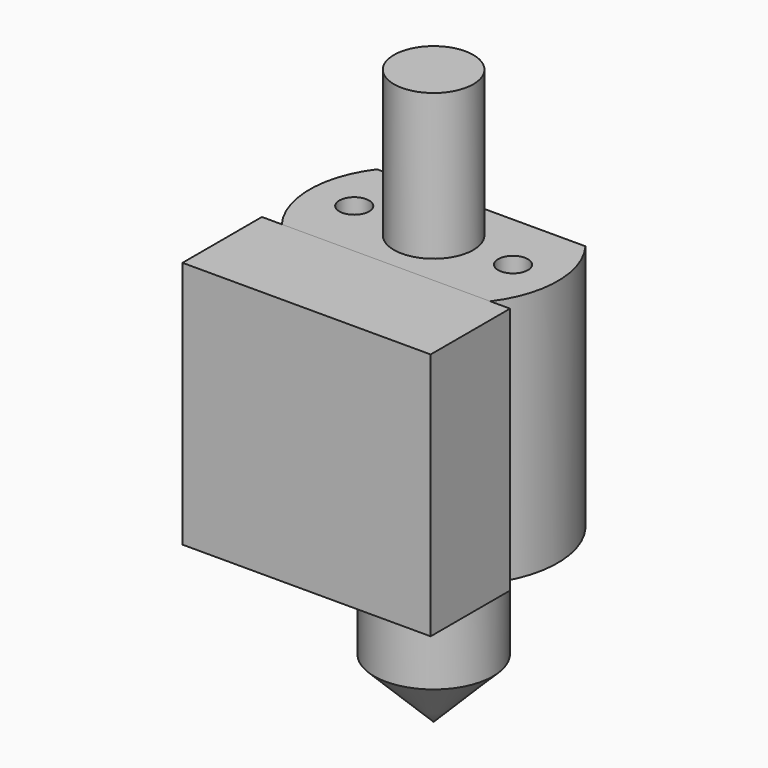
from build123d import *

# Parameters (mm, degrees)
F0_W     = 25
F0_H     = 25
F1_DEPTH = 10
F2_R     = 1.5
F3_DEPTH = 25
F4_R     = 4
F5_DEPTH = 14.7
F6_R     = 6
F7_DEPTH = 18.16
F8_SIZE  = 6


with BuildPart() as f1:
    # F0 (on Front) → F1 (new body)
    with BuildSketch(Plane.XZ):
        Rectangle(F0_W, F0_H)
    extrude(amount=F1_DEPTH)


with BuildPart() as f3:
    # F2 (on face) → F3 (new body)
    with BuildSketch(Plane.XY.offset(12.5)):
        with BuildLine():
            Line((10.5, 12), (-10.5, 12))
            ThreePointArc((-10.5, 12), (-12.5, 6), (-10.5, 0))
            Line((-10.5, 0), (10.5, 0))
            ThreePointArc((10.5, 0), (12.5, 6), (10.5, 12))
        make_face()
        with Locations((-8, 6)):
            Circle(F2_R, mode=Mode.SUBTRACT)
        with Locations((8, 6)):
            Circle(F2_R, mode=Mode.SUBTRACT)
    extrude(amount=-F3_DEPTH)

    # F4 (on face) → F5 (join)
    with BuildSketch(Plane.XY.offset(12.5)):
        with Locations((0, 6)):
            Circle(F4_R)
    extrude(amount=F5_DEPTH)

    # F6 (on face) → F7 (join)
    with BuildSketch(Plane(origin=(0, 0, -12.5), x_dir=(1, 0, 0), z_dir=(0, 0, -1))):
        with Locations((0, -6)):
            Circle(F6_R)
    extrude(amount=F7_DEPTH)

    # F8
    f8_edges = [f3.edges().sort_by_distance(p)[0] for p in [
        (-6, 6, -30.66),
    ]]
    chamfer(f8_edges, length=F8_SIZE)


solid = Compound([f1.part, f3.part])
